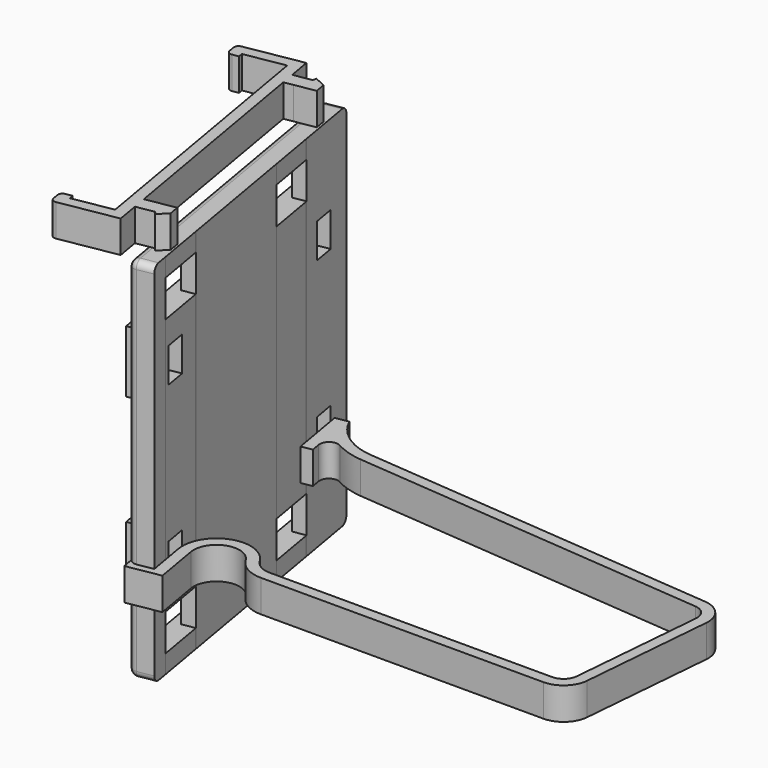
from build123d import *

# Parameters (mm, degrees)
F1_DEPTH      = 7
F4_DEPTH      = 40
F5_START      = 28
F5_DEPTH      = 8
F6_START      = -28
F6_DEPTH      = 8
F8_DEPTH      = 7
F9_R          = 1
F14_START     = -12
F14_DEPTH     = 13.5
F15_START     = 12
F15_DEPTH     = 13.5
F16_START     = -15
F16_DEPTH     = 7.5
F17_START     = 15
F17_DEPTH     = 7.5
F18_R         = 1.5
F19_T1_DEPTH  = 64.65
F19_T3_DEPTH  = 77
F19_T6_ANGLE  = 90
F19_T8_ANGLE  = 90
F19_T10_ANGLE = 90
F19_T12_ANGLE = 90


# Not quite as in the source:
# - a fillet or chamfer that OpenCascade refuses, or shapes differently, is made with other operations: its cross-section is extruded or revolved along the edge and cut away or added


with BuildPart() as f1:
    # F0 (on Top) → F1 (new body)
    with BuildSketch(Plane.XY):
        with BuildLine():
            ThreePointArc((9.2207398692, 3.4131401535), (11.7756352372, 0.9127995382), (15.2319324665, 0))
            Line((15.2319324665, 0), (76.7495216057, 0))
            ThreePointArc((76.7495216057, 0), (80.4695325258, 1.4488867265), (82.2295891023, 5.0321749984))
            Line((82.2295891023, 5.0321749984), (84.7345386464, 34.3749688426))
            ThreePointArc((84.7345386464, 34.3749688426), (83.460266269, 38.3869845015), (79.7222961513, 40.3228613409))
            Line((79.7222961513, 40.3228613409), (1.5067873354, 47))
            ThreePointArc((1.5067873354, 47), (-4.680872561, 49.2384235914), (-8.9188423513, 54.2720393123))
            Line((-8.9188423513, 54.2720393123), (-11.7267336042, 53.7870029843))
            Line((-11.7267336042, 53.7870029843), (-10.0245387921, 43.9329412419))
            Line((-10.0245387921, 43.9329412419), (-12.9807573606, 43.4222827904))
            Line((-12.9807573606, 43.4222827904), (-14.3135771745, 48.2153602302))
            Line((-14.3135771745, 48.2153602302), (-13.3501323588, 48.483267093))
            Line((-13.3501323588, 48.483267093), (-14.6829521727, 53.2763445327))
            Line((-14.6829521727, 53.2763445327), (-16.6537645211, 52.9359055703))
            Line((-16.6537645211, 52.9359055703), (-14.6111307467, 41.1110314795))
            Line((-14.6111307467, 41.1110314795), (-7.3191250573, 42.3706556404))
            Line((-7.3191250573, 42.3706556404), (-7.6610144107, 44.3498643501))
            ThreePointArc((-7.6610144107, 44.3498643501), (-6.8495844848, 46.3199757944), (-4.7223257599, 46.4405077186))
            ThreePointArc((-4.7223257599, 46.4405077186), (-1.8063622023, 45.2071338285), (1.3026455205, 44.6086978659))
            Line((1.3026455205, 44.6086978659), (79.5181543364, 37.9315592068))
            ThreePointArc((79.5181543364, 37.9315592068), (81.6250102525, 36.8404286082), (82.3432365123, 34.5791106576))
            Line((82.3432365123, 34.5791106576), (79.8382869683, 5.2363168133))
            ThreePointArc((79.8382869683, 5.2363168133), (78.8462550648, 3.2166452117), (76.7495216057, 2.3999999535))
            Line((76.7495216057, 2.3999999535), (15.2319324665, 2.3999999535))
            ThreePointArc((15.2319324665, 2.3999999535), (12.9606514072, 2.9998396561), (11.2817201484, 4.6429206485))
            ThreePointArc((11.2817201484, 4.6429206485), (2.3581944244, 7.7909157482), (-2.3649747724, -0.408526747))
            Line((-2.3649747724, -0.408526747), (-1.0032189227, -8.2917761409))
            Line((-1.0032189227, -8.2917761409), (-3.9594374912, -8.8024345924))
            Line((-3.9594374912, -8.8024345924), (-5.2922573051, -4.0093571526))
            Line((-5.2922573051, -4.0093571526), (-4.3288124894, -3.7414502898))
            Line((-4.3288124894, -3.7414502898), (-5.6616323033, 1.05162715))
            Line((-5.6616323033, 1.05162715), (-7.6324446517, 0.7111881875))
            Line((-7.6324446517, 0.7111881875), (-5.5898108773, -11.1136859033))
            Line((-5.5898108773, -11.1136859033), (1.7021948121, -9.8540617423))
            Line((1.7021948121, -9.8540617423), (0, 0))
            ThreePointArc((0, 0), (3.1913305584, 5.5401638829), (9.2207398692, 3.4131401535))
        make_face()
    extrude(amount=F1_DEPTH)


with BuildPart() as f4:
    # F3 (on offset) → F4 (new body, symmetric)
    with BuildSketch(Plane.XY.offset(25)):
        Polygon((-1.5986744983, -4.8446642331), (-3.3859790509, 5.5021005963), (-6.3421976194, 4.9914421448), (-7.6750174333, 9.7845195846), (-6.7115726176, 10.0524264473), (-8.0443924314, 14.8455038871), (-10.0152047799, 14.5050649247), (-6.5257054152, -5.6957616471), align=None)
        Polygon((-6.3421976194, 4.9914421448), (-3.3859790509, 5.5021005963), (-3.4115119731, 5.6499115225), (-6.2340305283, 5.162348468), (-7.4903146815, 9.6801888916), (-6.5268698658, 9.9480957544), (-7.9362253404, 15.0164102104), (-10.0407377021, 14.6528758509), (-10.0152047799, 14.5050649247), (-8.0443924314, 14.8455038871), (-6.7115726176, 10.0524264473), (-7.6750174333, 9.7845195846), align=None)
        Polygon((-0.9177965476, -8.7862890796), (-1.5986744983, -4.8446642331), (-6.5257054152, -5.6957616471), (-5.8448274645, -9.6373864935), align=None)
        Polygon((-6.2340305283, 5.162348468), (-3.4115119731, 5.6499115225), (-8.2372342395, 33.5861764125), (-13.1642651564, 32.7350789985), (-10.0407377021, 14.6528758509), (-7.9362253404, 15.0164102104), (-6.5268698658, 9.9480957544), (-7.4903146815, 9.6801888916), align=None)
        Polygon((-13.1642651564, 32.7350789985), (-8.2372342395, 33.5861764125), (-10.0245387921, 43.9329412419), (-12.9807573606, 43.4222827904), (-14.3135771745, 48.2153602302), (-13.3501323588, 48.483267093), (-14.6829521727, 53.2763445327), (-16.6537645211, 52.9359055703), align=None)
        Polygon((-12.9807573606, 43.4222827904), (-10.0245387921, 43.9329412419), (-10.0500717143, 44.0807521681), (-12.8725902695, 43.5931891136), (-14.1288744227, 48.1110295372), (-13.165429607, 48.3789364), (-14.5747850816, 53.447250856), (-16.6792974433, 53.0837164965), (-16.6537645211, 52.9359055703), (-14.6829521727, 53.2763445327), (-13.3501323588, 48.483267093), (-14.3135771745, 48.2153602302), align=None)
        Polygon((-12.8725902695, 43.5931891136), (-10.0500717143, 44.0807521681), (-12.4331444512, 57.8764386073), (-17.3601753681, 57.0253411934), (-16.6792974433, 53.0837164965), (-14.5747850816, 53.447250856), (-13.165429607, 48.3789364), (-14.1288744227, 48.1110295372), align=None)
    extrude(amount=F4_DEPTH, both=True)

    # F3 (on offset) → F5 (cut)
    with BuildSketch(Plane.XY.offset(25).offset(F5_START)):
        Polygon((-1.5986744983, -4.8446642331), (-3.3859790509, 5.5021005963), (-6.3421976194, 4.9914421448), (-7.6750174333, 9.7845195846), (-6.7115726176, 10.0524264473), (-8.0443924314, 14.8455038871), (-10.0152047799, 14.5050649247), (-6.5257054152, -5.6957616471), align=None)
        Polygon((-6.3421976194, 4.9914421448), (-3.3859790509, 5.5021005963), (-3.4115119731, 5.6499115225), (-6.2340305283, 5.162348468), (-7.4903146815, 9.6801888916), (-6.5268698658, 9.9480957544), (-7.9362253404, 15.0164102104), (-10.0407377021, 14.6528758509), (-10.0152047799, 14.5050649247), (-8.0443924314, 14.8455038871), (-6.7115726176, 10.0524264473), (-7.6750174333, 9.7845195846), align=None)
        Polygon((-13.1642651564, 32.7350789985), (-8.2372342395, 33.5861764125), (-10.0245387921, 43.9329412419), (-12.9807573606, 43.4222827904), (-14.3135771745, 48.2153602302), (-13.3501323588, 48.483267093), (-14.6829521727, 53.2763445327), (-16.6537645211, 52.9359055703), align=None)
        Polygon((-12.9807573606, 43.4222827904), (-10.0245387921, 43.9329412419), (-10.0500717143, 44.0807521681), (-12.8725902695, 43.5931891136), (-14.1288744227, 48.1110295372), (-13.165429607, 48.3789364), (-14.5747850816, 53.447250856), (-16.6792974433, 53.0837164965), (-16.6537645211, 52.9359055703), (-14.6829521727, 53.2763445327), (-13.3501323588, 48.483267093), (-14.3135771745, 48.2153602302), align=None)
    extrude(amount=F5_DEPTH, mode=Mode.SUBTRACT)

    # F3 (on offset) → F6 (cut)
    with BuildSketch(Plane.XY.offset(25).offset(F6_START)):
        Polygon((-1.5986744983, -4.8446642331), (-3.3859790509, 5.5021005963), (-6.3421976194, 4.9914421448), (-7.6750174333, 9.7845195846), (-6.7115726176, 10.0524264473), (-8.0443924314, 14.8455038871), (-10.0152047799, 14.5050649247), (-6.5257054152, -5.6957616471), align=None)
        Polygon((-6.3421976194, 4.9914421448), (-3.3859790509, 5.5021005963), (-3.4115119731, 5.6499115225), (-6.2340305283, 5.162348468), (-7.4903146815, 9.6801888916), (-6.5268698658, 9.9480957544), (-7.9362253404, 15.0164102104), (-10.0407377021, 14.6528758509), (-10.0152047799, 14.5050649247), (-8.0443924314, 14.8455038871), (-6.7115726176, 10.0524264473), (-7.6750174333, 9.7845195846), align=None)
        Polygon((-13.1642651564, 32.7350789985), (-8.2372342395, 33.5861764125), (-10.0245387921, 43.9329412419), (-12.9807573606, 43.4222827904), (-14.3135771745, 48.2153602302), (-13.3501323588, 48.483267093), (-14.6829521727, 53.2763445327), (-16.6537645211, 52.9359055703), align=None)
        Polygon((-12.9807573606, 43.4222827904), (-10.0245387921, 43.9329412419), (-10.0500717143, 44.0807521681), (-12.8725902695, 43.5931891136), (-14.1288744227, 48.1110295372), (-13.165429607, 48.3789364), (-14.5747850816, 53.447250856), (-16.6792974433, 53.0837164965), (-16.6537645211, 52.9359055703), (-14.6829521727, 53.2763445327), (-13.3501323588, 48.483267093), (-14.3135771745, 48.2153602302), align=None)
    extrude(amount=-F6_DEPTH, mode=Mode.SUBTRACT)

    # F13 (on face) → F14 (join)
    with BuildSketch(Plane.XY.offset(25).offset(F14_START)):
        Polygon((-8.289776023, -7.2330353446), (-6.3189636745, -6.8925963822), (-8.0211584866, 2.9614653601), (-9.9919708351, 2.6210263977), align=None)
        Polygon((-15.0963844862, 43.9201813351), (-16.7985792983, 53.7742430775), (-18.7693916468, 53.433804115), (-17.0671968347, 43.5797423727), align=None)
    extrude(amount=-F14_DEPTH)

    # F13 (on face) → F15 (join)
    with BuildSketch(Plane.XY.offset(25).offset(F15_START)):
        Polygon((-8.289776023, -7.2330353446), (-6.3189636745, -6.8925963822), (-8.0211584866, 2.9614653601), (-9.9919708351, 2.6210263977), align=None)
        Polygon((-15.0963844862, 43.9201813351), (-16.7985792983, 53.7742430775), (-18.7693916468, 53.433804115), (-17.0671968347, 43.5797423727), align=None)
    extrude(amount=F15_DEPTH)

    # F12 (on plane+point) → F16 (cut)
    with BuildSketch(Plane.XY.offset(25).offset(F16_START)):
        Polygon((-1.7716757996, -3.8431540105), (-2.5864213353, 0.8734346879), (-9.4842646007, -0.3181016885), (-8.7974822574, -4.2939072585), (-4.9248564436, -3.6249482301), (-4.5272702425, -4.3191565653), align=None)
        Polygon((-17.574903069, 46.5188704589), (-10.6770598036, 47.7104068352), (-11.4918053393, 52.4269955336), (-14.2473997822, 51.9509929787), (-14.3890595986, 51.1636350573), (-18.2616854124, 50.4946760289), align=None)
    extrude(amount=-F16_DEPTH, mode=Mode.SUBTRACT)

    # F12 (on plane+point) → F17 (cut)
    with BuildSketch(Plane.XY.offset(25).offset(F17_START)):
        Polygon((-1.7716757996, -3.8431540105), (-2.5864213353, 0.8734346879), (-9.4842646007, -0.3181016885), (-8.7974822574, -4.2939072585), (-4.9248564436, -3.6249482301), (-4.5272702425, -4.3191565653), align=None)
        Polygon((-17.574903069, 46.5188704589), (-10.6770598036, 47.7104068352), (-11.4918053393, 52.4269955336), (-14.2473997822, 51.9509929787), (-14.3890595986, 51.1636350573), (-18.2616854124, 50.4946760289), align=None)
    extrude(amount=F17_DEPTH, mode=Mode.SUBTRACT)

    # F18
    f18_edges = [f4.edges().sort_by_distance(p)[0] for p in [
        (-3.381312, -9.211838, -15),
        (-3.381312, -9.211838, 65),
        (-14.89666, 57.45089, 65),
        (-14.89666, 57.45089, -15),
    ]]
    fillet(f18_edges, radius=F18_R)

    # F19: fillet of radius 1.5 on 7 edges, made by hand

    # F19_s2 → F19_t1 (cut)
    with BuildSketch(Plane(origin=(-9.812840457, 56.806856093, 0), x_dir=(0, 0, 1), z_dir=(0.1702194812, -0.9854061742, 0))):
        with BuildLine():
            ThreePointArc((-13.5, 7.4), (-14.5606601718, 6.9606601718), (-15, 5.9))
            Line((-15, 5.9), (-15, 7.4))
            Line((-15, 7.4), (-13.5, 7.4))
        make_face()
        with BuildLine():
            ThreePointArc((63.5, 7.4), (64.5606601718, 6.9606601718), (65, 5.9))
            Line((65, 5.9), (65, 7.4))
            Line((65, 7.4), (63.5, 7.4))
        make_face()
    extrude(amount=F19_T1_DEPTH, mode=Mode.SUBTRACT)

    # F19_s4 → F19_t3 (cut)
    with BuildSketch(Plane.XY.offset(-13.5)):
        with BuildLine():
            ThreePointArc((-17.1048461463, 55.547231932), (-16.8524629912, 56.6671972117), (-15.8820661068, 57.2806704152))
            Line((-15.8820661068, 57.2806704152), (-17.3601753681, 57.0253411934))
            Line((-17.3601753681, 57.0253411934), (-17.1048461463, 55.547231932))
        make_face()
        with BuildLine():
            ThreePointArc((-4.3667182032, -9.3820572717), (-5.4866834829, -9.1296741166), (-6.1001566864, -8.1592772322))
            Line((-6.1001566864, -8.1592772322), (-5.8448274645, -9.6373864935))
            Line((-5.8448274645, -9.6373864935), (-4.3667182032, -9.3820572717))
        make_face()
    extrude(amount=F19_T3_DEPTH, mode=Mode.SUBTRACT)

    # F19_s5 → F19_t6 (revolve, cut)
    with BuildSketch(Plane.XY.offset(-13.5)):
        with BuildLine():
            ThreePointArc((-4.3667182032, -9.3820572717), (-5.4866834829, -9.1296741166), (-6.1001566864, -8.1592772322))
            Line((-6.1001566864, -8.1592772322), (-5.8448274645, -9.6373864935))
            Line((-5.8448274645, -9.6373864935), (-4.3667182032, -9.3820572717))
        make_face()
    revolve(axis=Axis((-6.1001566864, -8.1592772322, -13.5), (0.9854061742, 0.1702194812, 0)), revolution_arc=F19_T6_ANGLE, mode=Mode.SUBTRACT)

    # F19_s7 → F19_t8 (revolve, cut)
    with BuildSketch(Plane.XY.offset(63.5)):
        with BuildLine():
            ThreePointArc((-4.3667182032, -9.3820572717), (-5.4866834829, -9.1296741166), (-6.1001566864, -8.1592772322))
            Line((-6.1001566864, -8.1592772322), (-5.8448274645, -9.6373864935))
            Line((-5.8448274645, -9.6373864935), (-4.3667182032, -9.3820572717))
        make_face()
    revolve(axis=Axis((-6.1001566864, -8.1592772322, 63.5), (-0.9854061742, -0.1702194812, 0)), revolution_arc=F19_T8_ANGLE, mode=Mode.SUBTRACT)

    # F19_s9 → F19_t10 (revolve, cut)
    with BuildSketch(Plane(origin=(-9.812840457, 56.806856093, 0), x_dir=(0, 0, 1), z_dir=(0.1702194812, -0.9854061742, 0))):
        with BuildLine():
            ThreePointArc((-13.5, 7.4), (-14.5606601718, 6.9606601718), (-15, 5.9))
            Line((-15, 5.9), (-15, 7.4))
            Line((-15, 7.4), (-13.5, 7.4))
        make_face()
    revolve(axis=Axis((-17.1048461463, 55.547231932, -13.5), (0.9854061742, 0.1702194812, 0)), revolution_arc=F19_T10_ANGLE, mode=Mode.SUBTRACT)

    # F19_s11 → F19_t12 (revolve, cut)
    with BuildSketch(Plane(origin=(-9.812840457, 56.806856093, 0), x_dir=(0, 0, 1), z_dir=(0.1702194812, -0.9854061742, 0))):
        with BuildLine():
            ThreePointArc((63.5, 7.4), (64.5606601718, 6.9606601718), (65, 5.9))
            Line((65, 5.9), (65, 7.4))
            Line((65, 7.4), (63.5, 7.4))
        make_face()
    revolve(axis=Axis((-17.1048461463, 55.547231932, 63.5), (-0.9854061742, -0.1702194812, 0)), revolution_arc=F19_T12_ANGLE, mode=Mode.SUBTRACT)


with BuildPart() as f8:
    # F7 (on face) → F8 (new body)
    with BuildSketch(Plane.XY.offset(65)):
        Polygon((-21.364930769, -11.4373824566), (-7.9634067994, -9.1223975122), (-8.8145042055, -4.1953666411), (-9.3480890158, -1.1064266278), (-17.711078654, 47.3071953982), (-18.2446634643, 50.3961354115), (-19.0957608703, 55.3231662826), (-32.4972848399, 53.0081813382), (-31.9185386038, 49.6578003458), (-29.5535637856, 50.0663271007), (-29.7237832668, 51.051733275), (-21.0522089336, 52.5496647096), (-10.7369083725, -7.165949449), (-19.4084827058, -8.6638808836), (-19.578702187, -7.6784747094), (-21.9436770051, -8.0870014642), align=None)
        Polygon((-16.2738511158, 50.7365743739), (-15.7402663055, 47.6476343607), (-11.3059385215, 48.4136220261), (-11.7144652764, 50.7785968442), (-14.1613789509, 51.8643712577), (-14.3030387674, 51.0770133363), align=None)
        Polygon((-7.3772766673, -0.7659876654), (-6.843691857, -3.8549276787), (-4.8728795085, -3.5144887163), (-4.4752933075, -4.2086970515), (-2.5344221283, -2.3649748182), (-2.9429488832, 0), align=None)
        Polygon((-9.3480890158, -1.1064266278), (-8.8145042055, -4.1953666411), (-6.843691857, -3.8549276787), (-7.3772766673, -0.7659876654), align=None)
        Polygon((-18.2446634643, 50.3961354115), (-17.711078654, 47.3071953982), (-15.7402663055, 47.6476343607), (-16.2738511158, 50.7365743739), align=None)
    extrude(amount=F8_DEPTH)

    # F9
    f9_edges = [f8.edges().sort_by_distance(p)[0] for p in [
        (-21.364931, -11.437382, 68.5),
        (-21.943677, -8.087001, 68.5),
        (-32.497285, 53.008181, 68.5),
        (-31.918539, 49.6578, 68.5),
    ]]
    fillet(f9_edges, radius=F9_R)


solid = Compound([f1.part, f4.part, f8.part])
